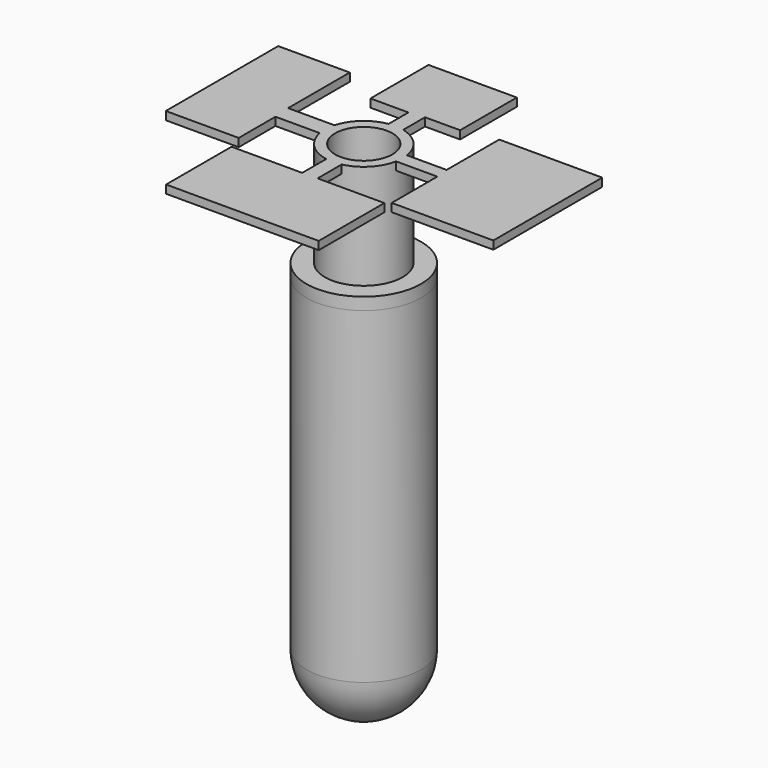
from build123d import *

# Parameters (mm, degrees)
F0_R      = 7
F1_DEPTH  = 7
F2_R      = 6.99999
F5_DEPTH  = 40
F6_R      = 7
F6_R_2    = 5.75
F7_DEPTH  = 1.5
F8_R      = 4.75
F8_R_2    = 3.5
F9_DEPTH  = 12.8
F11_DEPTH = 1


# Not quite as in the source:
# - a fillet or chamfer is up to 0.001 mm smaller than in the source, because OpenCascade refuses the exact size


with BuildPart() as f1:
    # F0 (on Top) → F1 (new body)
    with BuildSketch(Plane.XY):
        Circle(F0_R)
    extrude(amount=-F1_DEPTH)

    # F2 (radius 7 in the source; OpenCascade refuses exactly that, so slightly less here)
    f2_edges = [f1.edges().sort_by_distance(p)[0] for p in [
        (-7, 0, -7),
    ]]
    fillet(f2_edges, radius=F2_R)

    # F3 (on face) → F4 (revolve, cut)
    with BuildSketch(Plane.XY):
        with BuildLine():
            Line((-5.75, 0), (5.75, 0))
            ThreePointArc((5.75, 0), (0, 5.75), (-5.75, 0))
        make_face()
    revolve(axis=Axis((0, 0, 0), (1, 0, 0)), mode=Mode.SUBTRACT)

    # F5 (add): a face of the model
    f5_faces = [f1.faces().sort_by_distance(p)[0] for p in [
        (-6.8020101013, 0, 0),
    ]]
    extrude(f5_faces, amount=F5_DEPTH)

    # F6 (on face) → F7 (join)
    with BuildSketch(Plane.XY.offset(40)):
        Circle(F6_R)
        Circle(F6_R_2, mode=Mode.SUBTRACT)
        Circle(F6_R_2)
    extrude(amount=F7_DEPTH)

    # F8 (on face) → F9 (join)
    with BuildSketch(Plane.XY.offset(41.5)):
        Circle(F8_R)
        Circle(F8_R_2, mode=Mode.SUBTRACT)
    extrude(amount=F9_DEPTH)

    # F10 (on face) → F11 (join)
    with BuildSketch(Plane.XY.offset(54.3)):
        with BuildLine():
            ThreePointArc((-4.6668358831, -0.8849535807), (-4.7461193146, 0.1919673186), (-4.5801202528, 1.2589672237))
            Line((-4.5801202528, 1.2589672237), (-10.254695956, 1.2589672237))
            Line((-10.254695956, 1.2589672237), (-10.254695956, 10.6798189955))
            Line((-10.254695956, 10.6798189955), (-18.9986647217, 10.6798189955))
            Line((-18.9986647217, 10.6798189955), (-18.9986647217, -6.4948128273))
            Line((-18.9986647217, -6.4948128273), (-10.0838066189, -6.4948128273))
            Line((-10.0838066189, -6.4948128273), (-10.0838066189, -0.8849535807))
            Line((-10.0838066189, -0.8849535807), (-4.6668358831, -0.8849535807))
        make_face()
        with BuildLine():
            Line((-0.7236261107, 7.7295311092), (-0.7236261107, 4.6945569814))
            ThreePointArc((-0.7236261107, 4.6945569814), (0.2079220104, 4.7454471273), (1.1314493255, 4.6132767556))
            Line((1.1314493255, 4.6132767556), (1.1314493255, 7.9441230255))
            Line((1.1314493255, 7.9441230255), (5.4202612606, 7.9441230255))
            Line((5.4202612606, 7.9441230255), (5.4202612606, 16.6028177181))
            Line((5.4202612606, 16.6028177181), (-5.3641636993, 16.6028177181))
            Line((-5.3641636993, 16.6028177181), (-5.3641636993, 7.7295311092))
            Line((-5.3641636993, 7.7295311092), (-0.7236261107, 7.7295311092))
        make_face()
        with BuildLine():
            Line((9.5364480238, 0.7383154319), (4.6922692083, 0.7383154319))
            ThreePointArc((4.6922692083, 0.7383154319), (4.7355453086, 0.3702845262), (4.75, 0))
            ThreePointArc((4.75, 0), (4.7285644054, -0.4507534407), (4.6644510887, -0.8974386001))
            Line((4.6644510887, -0.8974386001), (9.7088032833, -0.8974386001))
            Line((9.7088032833, -0.8974386001), (9.7088032833, -7.8623809823))
            Line((9.7088032833, -7.8623809823), (22.1269458032, -7.8623809823))
            Line((22.1269458032, -7.8623809823), (22.1269458032, -5.6407864176))
            Line((22.1269458032, -5.6407864176), (22.1269458032, 8.7704470205))
            Line((22.1269458032, 8.7704470205), (9.5364480238, 8.7704470205))
            Line((9.5364480238, 8.7704470205), (9.5364480238, 0.7383154319))
        make_face()
        with BuildLine():
            ThreePointArc((1.0145288717, -4.6403912732), (0.0864892709, -4.7492125248), (-0.8448971996, -4.6742538145))
            Line((-0.8448971996, -4.6742538145), (-0.8448971996, -8.3471687661))
            Line((-0.8448971996, -8.3471687661), (-9.48290206, -8.3471687661))
            Line((-9.48290206, -8.3471687661), (-9.48290206, -18.3443419333))
            Line((-9.48290206, -18.3443419333), (9.1727929611, -18.3443419333))
            Line((9.1727929611, -18.3443419333), (9.1727929611, -8.3204683216))
            Line((9.1727929611, -8.3204683216), (1.0145288717, -8.3204683216))
            Line((1.0145288717, -8.3204683216), (1.0145288717, -4.6403912732))
        make_face()
    extrude(amount=-F11_DEPTH)


solid = f1.part
